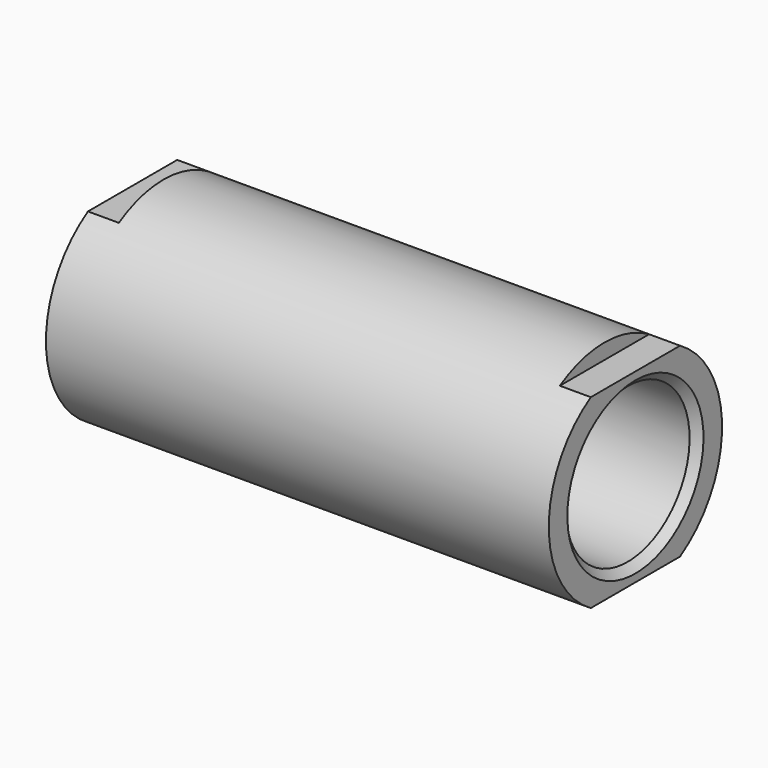
from build123d import *

# Parameters (mm, degrees)
F2_R     = 1
F3_SIZE  = 1
F5_DEPTH = 4
F7_DEPTH = 4


with BuildPart() as f1:
    # F0 (on Front) → F1 (revolve)
    with BuildSketch(Plane.XZ):
        Polygon((-32, 14), (-32, 10), (-17, 10), (-17, 8), (18, 8), (18, 10), (33, 10), (33, 14), align=None)
    revolve(axis=Axis((4.3690800667, 0, 0), (-1, 0, 0)))

    # F2
    f2_edges = [f1.edges().sort_by_distance(p)[0] for p in [
        (18, 0, -10),
        (-17, 0, -10),
    ]]
    fillet(f2_edges, radius=F2_R)

    # F3
    f3_edges = [f1.edges().sort_by_distance(p)[0] for p in [
        (-32, 0, -10),
        (33, 0, -10),
    ]]
    chamfer(f3_edges, length=F3_SIZE)

    # F4 (on face) → F5 (cut)
    with BuildSketch(Plane(origin=(-32, 0, 0), x_dir=(0, -1, 0), z_dir=(-1, 0, 0))):
        with BuildLine():
            Line((0, 14), (-10, 14))
            Line((-10, 14), (-10, 12))
            Line((-10, 12), (-7.2111025509, 12))
            ThreePointArc((-7.2111025509, 12), (-3.7416573868, 13.4907375632), (0, 14))
        make_face()
        with BuildLine():
            ThreePointArc((7.2111025509, 12), (3.7416573868, 13.4907375632), (0, 14))
            ThreePointArc((0, 14), (-3.7416573868, 13.4907375632), (-7.2111025509, 12))
            Line((-7.2111025509, 12), (7.2111025509, 12))
        make_face()
        with BuildLine():
            Line((10, 14), (0, 14))
            ThreePointArc((0, 14), (3.7416573868, 13.4907375632), (7.2111025509, 12))
            Line((7.2111025509, 12), (10, 12))
            Line((10, 12), (10, 14))
        make_face()
        with BuildLine():
            ThreePointArc((0, -14), (-3.7416573868, -13.4907375632), (-7.2111025509, -12))
            Line((-7.2111025509, -12), (-10, -12))
            Line((-10, -12), (-10, -14))
            Line((-10, -14), (0, -14))
        make_face()
        with BuildLine():
            Line((7.2111025509, -12), (-7.2111025509, -12))
            ThreePointArc((-7.2111025509, -12), (-3.7416573868, -13.4907375632), (0, -14))
            ThreePointArc((0, -14), (3.7416573868, -13.4907375632), (7.2111025509, -12))
        make_face()
        with BuildLine():
            Line((10, -12), (7.2111025509, -12))
            ThreePointArc((7.2111025509, -12), (3.7416573868, -13.4907375632), (0, -14))
            Line((0, -14), (10, -14))
            Line((10, -14), (10, -12))
        make_face()
    extrude(amount=-F5_DEPTH, mode=Mode.SUBTRACT)

    # F6 (on face) → F7 (cut)
    with BuildSketch(Plane.YZ.offset(33)):
        with BuildLine():
            ThreePointArc((7.2111025509, 12), (3.7416573868, 13.4907375632), (0, 14))
            ThreePointArc((0, 14), (-3.7416573868, 13.4907375632), (-7.2111025509, 12))
            Line((-7.2111025509, 12), (7.2111025509, 12))
        make_face()
        with BuildLine():
            Line((7.2111025509, -12), (-7.2111025509, -12))
            ThreePointArc((-7.2111025509, -12), (-3.7416573868, -13.4907375632), (0, -14))
            ThreePointArc((0, -14), (3.7416573868, -13.4907375632), (7.2111025509, -12))
        make_face()
    extrude(amount=-F7_DEPTH, mode=Mode.SUBTRACT)


solid = f1.part
